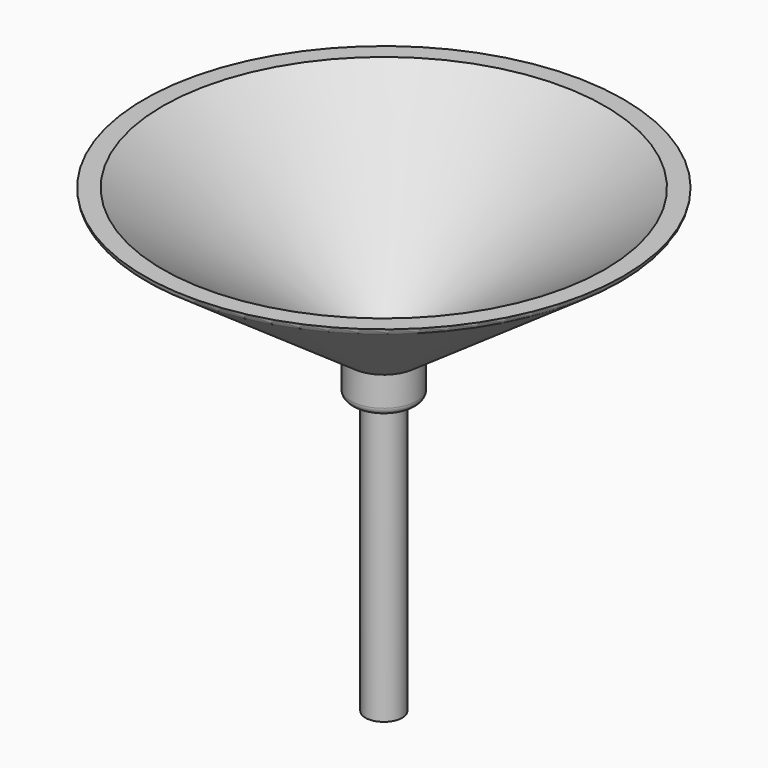
from build123d import *

# Parameters (mm, degrees)
F0_R       = 65
F0_R_2     = 60
F1_DEPTH   = 40
F2_R       = 3
F4_SIZE2   = 56
F4_SIZE    = 39
F5_DEPTH   = 10
F8_R       = 5
F8_R_2     = 3
F9_DEPTH   = 42
F10_OFFSET = 0.2
F11_DEPTH  = 40


# Not quite as in the source:
# - a fillet or chamfer that OpenCascade refuses, or shapes differently, is made with other operations: its cross-section is extruded or revolved along the edge and cut away or added


with BuildPart() as f1:
    # F0 (on Top) → F1 (new body)
    with BuildSketch(Plane.XY):
        Circle(F0_R)
        Circle(F0_R_2, mode=Mode.SUBTRACT)
        Circle(F0_R_2)
    extrude(amount=-F1_DEPTH)

    # F0 (on Top) → F3 section 0
    with BuildSketch(Plane.XY):
        Circle(F0_R_2)
    # F2 (on face) → F3 section 1
    with BuildSketch(Plane(origin=(0, 0, -40), x_dir=(1, 0, 0), z_dir=(0, 0, -1))):
        Circle(F2_R)
    loft(mode=Mode.SUBTRACT)

    # F4
    f4_edges = [f1.edges().sort_by_distance(p)[0] for p in [
        (-65, 0, -40),
    ]]
    f4_side = f1.faces().sort_by_distance((-65, 0, -20))[0]
    chamfer(f4_edges, length=F4_SIZE, length2=F4_SIZE2, reference=f4_side)

    # F5 (add): a face of the model
    f5_faces = [f1.faces().sort_by_distance(p)[0] for p in [
        (-8.7454415588, 0, -40),
    ]]
    extrude(f5_faces, amount=F5_DEPTH)

    # F6: fillet of radius 2 on 2 edges, made by hand

    # F6_s1 → F6_t2 (revolve, cut)
    with BuildSketch(Plane.XZ):
        with BuildLine():
            ThreePointArc((65, 0.0443648455), (64.7728472883, -0.8813848467), (64.1429875075, -1.5968479858))
            Line((64.1429875075, -1.5968479858), (65, -1))
            Line((65, -1), (65, 0.0443648455))
        make_face()
    revolve(axis=Axis((0, 0, -1), (0, 0, 1)), mode=Mode.SUBTRACT)

    # F6_s3 → F6_t4 (revolve, cut)
    with BuildSketch(Plane.XZ):
        with BuildLine():
            ThreePointArc((9, -48), (8.4142135624, -49.4142135624), (7, -50))
            Line((7, -50), (9, -50))
            Line((9, -50), (9, -48))
        make_face()
    revolve(axis=Axis((0, 0, -50), (0, 0, 1)), mode=Mode.SUBTRACT)


with BuildPart() as f9:
    # F8 (on offset) → F9 (new body)
    with BuildSketch(Plane.XY.offset(-85)):
        Circle(F8_R)
        Circle(F8_R_2, mode=Mode.SUBTRACT)
    extrude(amount=F9_DEPTH)


with BuildPart() as f1_1:
    add(f1.part)

    # F10: cut F9, made larger all round first
    f10_tool = offset(f9.part, amount=F10_OFFSET, kind=Kind.INTERSECTION, mode=Mode.PRIVATE)
    add(f10_tool, mode=Mode.SUBTRACT)


with BuildPart() as f9_1:
    add(f9.part)

    # F11 (add): a face of the model
    f11_faces = [f9_1.faces().sort_by_distance(p)[0] for p in [
        (-4.8585786438, 0, -85),
    ]]
    extrude(f11_faces, amount=F11_DEPTH)


solid = Compound([f1_1.part, f9_1.part])
